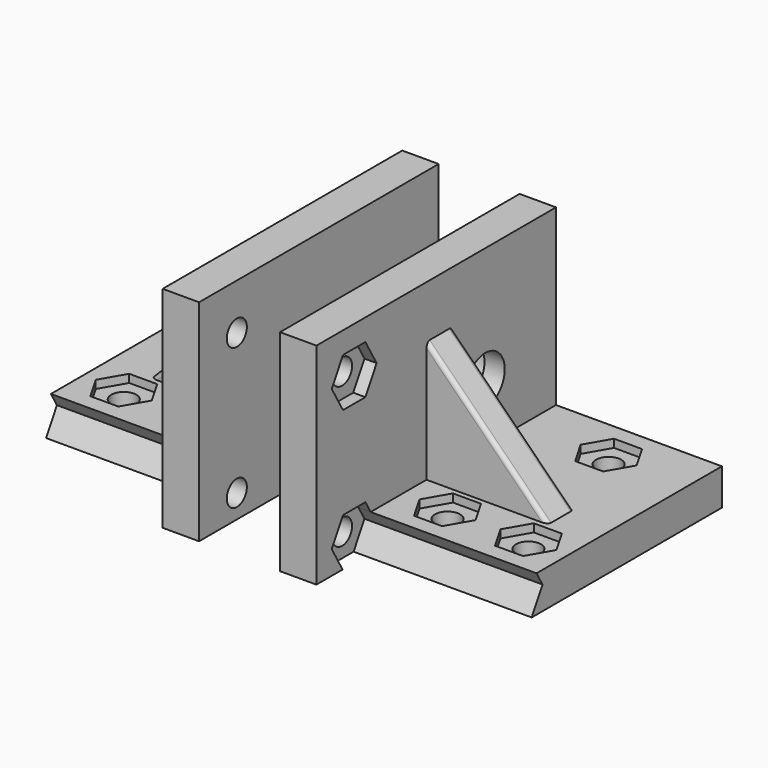
from build123d import *

# Parameters (mm, degrees)
F1_DEPTH      = 19
F1_DEPTH_BACK = 18
F2_DEPTH      = 2
F2_DEPTH_BACK = 2
F3_R          = 1.55
F4_DEPTH      = 26
F6_DEPTH      = 22
F7_DEPTH      = 20.5
F8_R          = 1.55
F9_DEPTH      = 1
F10_DEPTH     = 6
F11_R         = 0.5
F3_R_2        = 3
F12_DEPTH     = 6
F3_R_3        = 4
F3_R_4        = 2.4
F13_DEPTH     = 2


with BuildPart() as f1:
    # F0 (on Front) → F1 (new body, two sides)
    with BuildSketch(Plane.XZ) as f1_sk:
        Polygon((0, 26), (0, 0), (25, 0), (25, 4.5), (19.5, 4.5), (4.5, 4.5), (4.5, 19.5), (4.5, 26), align=None)
    extrude(amount=F1_DEPTH)
    extrude(f1_sk.sketch, amount=-F1_DEPTH_BACK)

    # F0 (on Front) → F2 (join, two sides)
    with BuildSketch(Plane.XZ) as f2_sk:
        Polygon((19.5, 4.5), (4.5, 19.5), (4.5, 4.5), align=None)
    extrude(amount=F2_DEPTH)
    extrude(f2_sk.sketch, amount=-F2_DEPTH_BACK)

    # F3 (on face) → F4 (cut)
    with BuildSketch(Plane(origin=(0, 0, 0), x_dir=(0, -1, 0), z_dir=(-1, 0, 0))):
        with Locations((13.17, 2.9)):
            Circle(F3_R)
        with Locations((13.17, 20.32)):
            Circle(F3_R)
    extrude(amount=-F4_DEPTH, mode=Mode.SUBTRACT)

    # F5 (on face) → F6 (cut)
    with BuildSketch(Plane.YZ.offset(25)):
        Polygon((-14.9020508076, 17.32), (-11.4379491924, 17.32), (-9.7058983849, 20.32), (-11.4379491924, 23.32), (-14.9020508076, 23.32), (-16.6341016151, 20.32), align=None)
        Polygon((-14.9020508076, -0.1), (-11.4379491924, -0.1), (-11.3802141655, 0), (-14.5227368921, 0), (-14.9597858345, 0), align=None)
        Polygon((-14.5227368921, 4.5), (-10.6296588156, 4.5), (-11.4379491924, 5.9), (-14.9020508076, 5.9), (-15.7103411844, 4.5), align=None)
        with BuildLine():
            Line((-16.6341016151, 2.9), (-14.9597858345, 0))
            Line((-14.9597858345, 0), (-14.5227368921, 0))
            Line((-14.5227368921, 0), (-14.5227368921, 2.1432947068))
            ThreePointArc((-14.5227368921, 2.1432947068), (-14.72, 2.9), (-14.5227368921, 3.6567052932))
            Line((-14.5227368921, 3.6567052932), (-14.5227368921, 4.5))
            Line((-14.5227368921, 4.5), (-15.7103411844, 4.5))
            Line((-15.7103411844, 4.5), (-16.6341016151, 2.9))
        make_face()
        with BuildLine():
            Line((-14.5227368921, 0), (-11.3802141655, 0))
            Line((-11.3802141655, 0), (-9.7058983849, 2.9))
            Line((-9.7058983849, 2.9), (-10.6296588156, 4.5))
            Line((-10.6296588156, 4.5), (-14.5227368921, 4.5))
            Line((-14.5227368921, 4.5), (-14.5227368921, 3.6567052932))
            ThreePointArc((-14.5227368921, 3.6567052932), (-12.7790026744, 4.3998736918), (-11.62, 2.9))
            ThreePointArc((-11.62, 2.9), (-12.7790026744, 1.4001263082), (-14.5227368921, 2.1432947068))
            Line((-14.5227368921, 2.1432947068), (-14.5227368921, 0))
        make_face()
    extrude(amount=-F6_DEPTH, mode=Mode.SUBTRACT)

    # F7 (cut): a face of the model
    f7_faces = [f1.faces().sort_by_distance(p)[0] for p in [
        (25, -17.4312907, 2.1162889805),
    ]]
    extrude(f7_faces, amount=-F7_DEPTH, mode=Mode.SUBTRACT)

    # F8 (on face) → F9 (cut)
    with BuildSketch(Plane.XY.offset(4.5)):
        Polygon((8.2679491924, -8.6296588156), (11.7320508076, -8.6296588156), (13.4641016151, -5.6296588156), (11.7320508076, -2.6296588156), (8.2679491924, -2.6296588156), (6.5358983849, -5.6296588156), align=None)
        with Locations((10, -5.6296588156)):
            Circle(F8_R, mode=Mode.SUBTRACT)
        Polygon((18.2679491924, -8.6296588156), (21.7320508076, -8.6296588156), (23.4641016151, -5.6296588156), (21.7320508076, -2.6296588156), (18.2679491924, -2.6296588156), (16.5358983849, -5.6296588156), align=None)
        with Locations((20, -5.6296588156)):
            Circle(F8_R, mode=Mode.SUBTRACT)
        Polygon((16.7320508076, 16), (13.2679491924, 16), (11.5358983849, 13), (13.2679491924, 10), (16.7320508076, 10), (18.4641016151, 13), align=None)
        with Locations((15, 13)):
            Circle(F8_R, mode=Mode.SUBTRACT)
        with Locations((10, -5.6296588156)):
            Circle(F8_R)
        with Locations((20, -5.6296588156)):
            Circle(F8_R)
        with Locations((15, 13)):
            Circle(F8_R)
    extrude(amount=-F9_DEPTH, mode=Mode.SUBTRACT)

    # F8 (on face) → F10 (cut)
    with BuildSketch(Plane.XY.offset(4.5)):
        with Locations((10, -5.6296588156)):
            Circle(F8_R)
        with Locations((20, -5.6296588156)):
            Circle(F8_R)
        with Locations((15, 13)):
            Circle(F8_R)
    extrude(amount=-F10_DEPTH, mode=Mode.SUBTRACT)

    # F11
    f11_edges = [f1.edges().sort_by_distance(p)[0] for p in [
        (12, -2, 12),
        (12, 2, 12),
    ]]
    fillet(f11_edges, radius=F11_R)

    # F3 (on face) → F12 (cut)
    with BuildSketch(Plane(origin=(0, 0, 0), x_dir=(0, -1, 0), z_dir=(-1, 0, 0))):
        with Locations((-7.08, 11.61)):
            Circle(F3_R_2)
    extrude(amount=-F12_DEPTH, mode=Mode.SUBTRACT)

    # F3 (on face) → F13 (cut)
    with BuildSketch(Plane(origin=(0, 0, 0), x_dir=(0, -1, 0), z_dir=(-1, 0, 0))):
        with Locations((-7.08, 11.61)):
            Circle(F3_R_3)
        with Locations((-7.08, 11.61)):
            Circle(F3_R_2, mode=Mode.SUBTRACT)
        with Locations((4, 11.61)):
            Circle(F3_R_4)
    extrude(amount=-F13_DEPTH, mode=Mode.SUBTRACT)


with BuildPart() as f15_1:
    # F15: instance of F1
    add(f1.part.mirror(Plane(origin=(-5, 0, 0), x_dir=(0, -1, 0), z_dir=(-1, 0, 0))))


solid = Compound([f1.part, f15_1.part])
